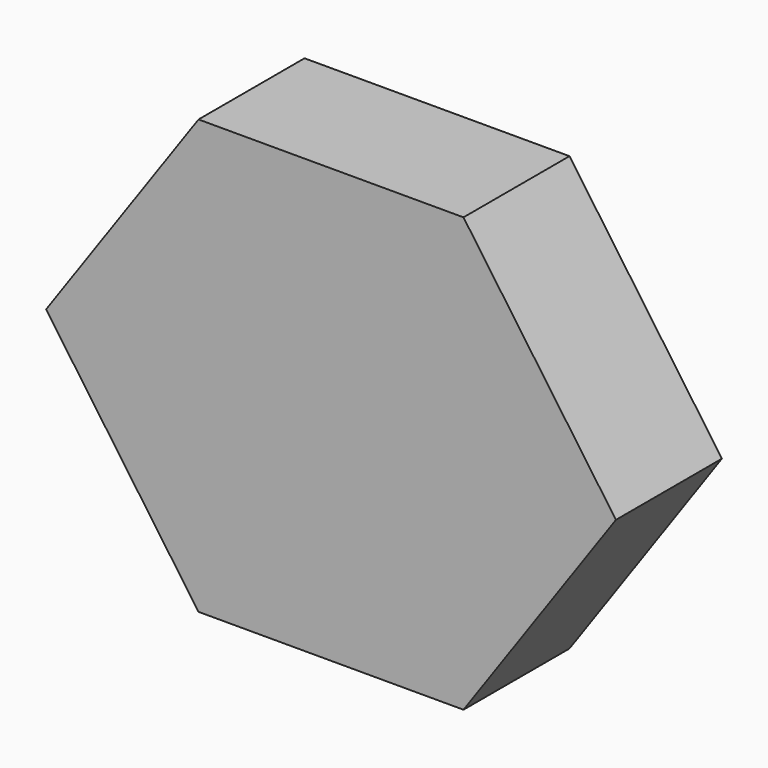
from build123d import *

# Parameters (mm, degrees)
F1_DEPTH = 12.7


# Not quite as in the source:
# - the program builds the solid bodies; features that only make, move or delete a surface that nothing else refers to are left out


with BuildPart() as f1:
    # F0 (on Front) → F1 (new body)
    with BuildSketch(Plane.XZ):
        Polygon((7.7044456086, 20.7762341559), (-17.6955543914, 20.7762341559), (-32.3074705662, 0), (-17.6955543914, -20.7762341559), (7.7044456086, -20.7762341559), (22.3163617834, 0), align=None)
    extrude(amount=F1_DEPTH)


solid = f1.part
